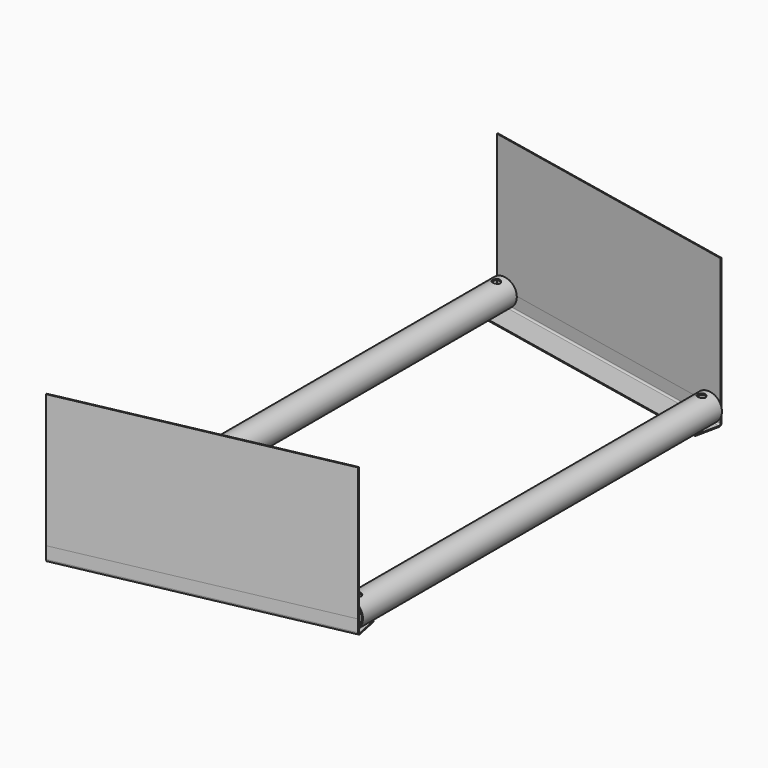
from build123d import *

# Parameters (mm, degrees)
F0_R      = 16
F0_R_2    = 14.4
F1_DEPTH  = 322.5
F2_R      = 16
F2_R_2    = 14.4
F3_DEPTH  = 262.5
F5_DEPTH  = 156
F7_DEPTH  = 320
F9_R      = 4.5
F10_DEPTH = 18


with BuildPart() as f1:
    # F0 (on Front) → F1 (new body, symmetric)
    with BuildSketch(Plane.XZ):
        with Locations((-144, 0)):
            Circle(F0_R)
        with Locations((-144, 0)):
            Circle(F0_R_2, mode=Mode.SUBTRACT)
    extrude(amount=F1_DEPTH, both=True)


with BuildPart() as f3:
    # F2 (on Front) → F3 (new body, symmetric)
    with BuildSketch(Plane.XZ):
        with Locations((144, 0)):
            Circle(F2_R)
        with Locations((144, 0)):
            Circle(F2_R_2, mode=Mode.SUBTRACT)
    extrude(amount=F3_DEPTH, both=True)


with BuildPart() as f5:
    # F4 (on Top) → F5 (new body)
    with BuildSketch(Plane.XY):
        Polygon((156.7568603372, -264.5), (-156.6057600682, -329.3372434071), (-156.3626204054, -330.5123532336), (157, -265.6751098265), align=None)
    extrude(amount=F5_DEPTH)

    # F6 (on face) → F7 (join)
    with BuildSketch(Plane(origin=(-215.5216002673, -44.5931503826, 0), x_dir=(0.2026163856, -0.9792581888, 0), z_dir=(-0.9792581888, -0.2026163856, 0))):
        with BuildLine():
            Line((291.9752993958, 0), (290.7752993958, 0))
            Line((290.7752993958, 0), (290.7752993958, -14))
            ThreePointArc((290.7752993958, -14), (290.1895129582, -15.4142135624), (288.7752993958, -16))
            Line((288.7752993958, -16), (260.7752993958, -16))
            Line((260.7752993958, -16), (260.7752993958, -17.2))
            Line((260.7752993958, -17.2), (288.9752993958, -17.2))
            ThreePointArc((288.9752993958, -17.2), (291.0966197394, -16.3213203436), (291.9752993958, -14.2))
            Line((291.9752993958, -14.2), (291.9752993958, 0))
        make_face()
    extrude(amount=-F7_DEPTH)


with BuildPart() as f8_1:
    # F8: instance of F5
    add(f5.part.mirror(Plane.XZ))


with BuildPart() as f10_tool:
    # F9 (on Top) → F10 (new body, symmetric)
    with BuildSketch(Plane.XY):
        with Locations((-143.0109928395, -311.2066596619)):
            Circle(F9_R)
        with Locations((144.7568603372, -251.6651791975)):
            Circle(F9_R)
        with Locations((144.7568603372, 251.6651791975)):
            Circle(F9_R)
        with Locations((-143.0109928395, 311.2066596619)):
            Circle(F9_R)
    extrude(amount=F10_DEPTH, both=True)


with BuildPart() as f1_1:
    add(f1.part)

    # F10: cut by f10_tool
    add(f10_tool.part, mode=Mode.SUBTRACT)


with BuildPart() as f3_1:
    add(f3.part)

    # F10: cut by f10_tool
    add(f10_tool.part, mode=Mode.SUBTRACT)


with BuildPart() as f5_1:
    add(f5.part)

    # F10: cut by f10_tool
    add(f10_tool.part, mode=Mode.SUBTRACT)


with BuildPart() as f8_1_1:
    add(f8_1.part)

    # F10: cut by f10_tool
    add(f10_tool.part, mode=Mode.SUBTRACT)


solid = Compound([f1_1.part, f3_1.part, f5_1.part, f8_1_1.part])
